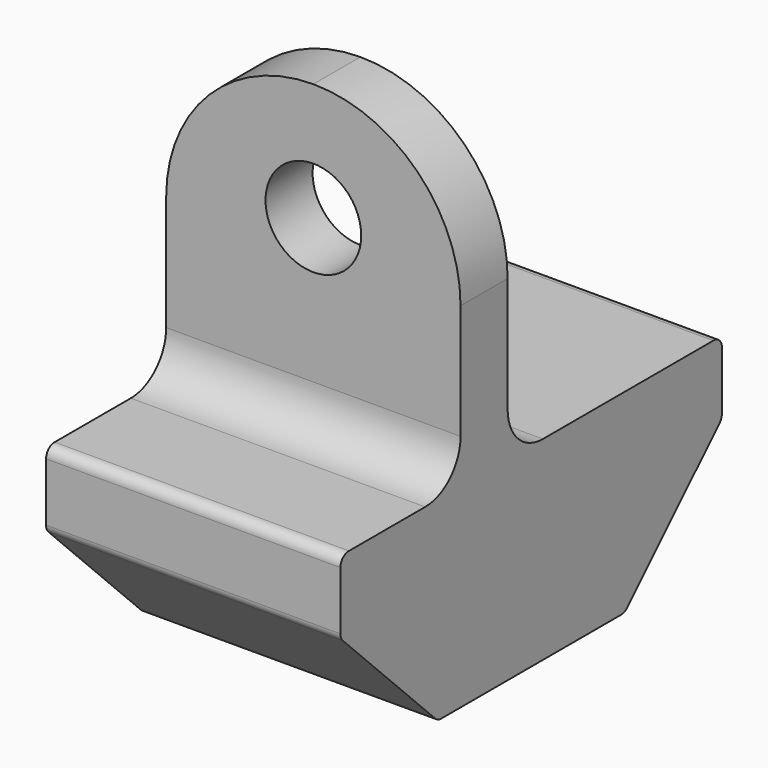
from build123d import *

# Parameters (mm, degrees)
F2_DEPTH = 5
F3_R     = 1.5
F4_R     = 4.99999
F6_D     = 3.25


# Not quite as in the source:
# - a fillet or chamfer is up to 0.001 mm smaller than in the source, because OpenCascade refuses the exact size


with BuildPart() as f2:
    # F1 (on Right) → F2 (new body, symmetric)
    with BuildSketch(Plane.YZ):
        with BuildLine():
            Line((-4.5, 12.592475), (-7.7353845436, 12.592475))
            ThreePointArc((-7.7353845436, 12.592475), (-7.9922437092, 12.4953707173), (-8.099967, 12.242781))
            Line((-8.099967, 12.242781), (-8.099967, 10.260188))
            ThreePointArc((-8.099967, 10.260188), (-8.0733249886, 10.126249564), (-7.9974549592, 10.0127020408))
            Line((-7.9974549828, 10.0127020172), (-4.0719369828, 6.0871840172))
            ThreePointArc((-4.0719369592, 6.0871840408), (-3.958389436, 6.0113140114), (-3.824451, 5.984672))
            Line((-3.824451, 5.984672), (-0.949996, 5.984672))
            Line((-0.949996, 5.984672), (0.949996, 5.984672))
            Line((0.949996, 5.984672), (3.824451, 5.984672))
            ThreePointArc((3.824451, 5.984672), (3.958389436, 6.0113140114), (4.0719369592, 6.0871840408))
            Line((4.0719369828, 6.0871840172), (7.9974549828, 10.0127020172))
            ThreePointArc((7.9974549592, 10.0127020408), (8.0733249886, 10.126249564), (8.099967, 10.260188))
            Line((8.099967, 10.260188), (8.099967, 12.242781))
            ThreePointArc((8.099967, 12.242781), (7.9922437092, 12.4953707173), (7.7353845436, 12.592475))
            Line((7.7353845436, 12.592475), (4.5, 12.592475))
            Line((4.5, 12.592475), (-1, 12.592475))
            Line((-1, 12.592475), (-1, 22.99994))
            Line((-1, 22.99994), (-3, 22.99994))
            Line((-3, 22.99994), (-3, 12.592475))
            Line((-3, 12.592475), (-4.5, 12.592475))
        make_face()
    extrude(amount=F2_DEPTH, both=True)

    # F3
    f3_edges = [f2.edges().sort_by_distance(p)[0] for p in [
        (0, -3, 12.592475),
        (0, -1, 12.592475),
    ]]
    fillet(f3_edges, radius=F3_R)

    # F4 (radius 5 in the source; OpenCascade refuses exactly that, so slightly less here)
    f4_edges = [f2.edges().sort_by_distance(p)[0] for p in [
        (5, -2, 22.99994),
        (-5, -2, 22.99994),
    ]]
    fillet(f4_edges, radius=F4_R)

    # F6 (through all)
    with Locations(Plane(origin=(0, -1, 0), x_dir=(-1, 0, 0), z_dir=(0, 1, 0))):
        with Locations((0, 18.99994)):
            Hole(F6_D / 2)


solid = f2.part
